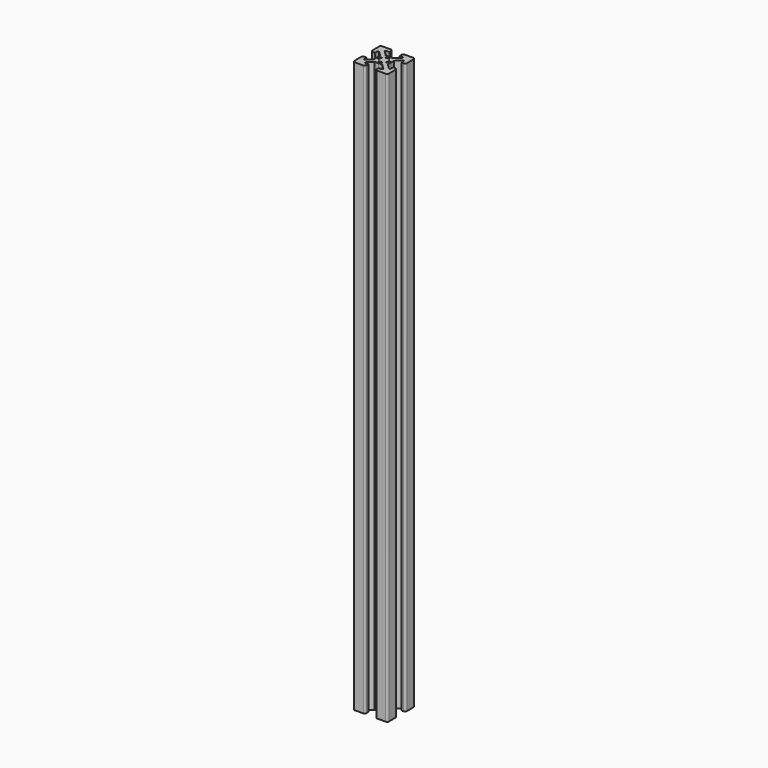
from build123d import *

# Parameters (mm, degrees)
F1_DEPTH = 330
F2_R     = 1
F3_R     = 0.5
F4_R     = 0.1


with BuildPart() as f1:
    # F0 (on Top) → F1 (new body)
    with BuildSketch(Plane.XY):
        with BuildLine():
            Line((-0.025, 4.0583112277), (-2.2905442747, 4.0583112277))
            Line((-2.2905442747, 4.0583112277), (-5.8640526549, 7.6318196079))
            Line((-5.8640526549, 7.6318196079), (-3, 7.6318196079))
            Line((-3, 7.6318196079), (-3, 10))
            Line((-3, 10), (-10, 10))
            Line((-10, 10), (-10, 3))
            Line((-10, 3), (-7.6318196079, 3))
            Line((-7.6318196079, 3), (-7.6318196079, 5.8640526549))
            Line((-7.6318196079, 5.8640526549), (-4, 2.232233047))
            Line((-4, 2.232233047), (-4, 0.025))
            Line((-4, 0.025), (-2.8230957687, 0.025))
            Line((-2.8230957687, 0.025), (-2.8230957687, 0.7926485917))
            Line((-2.8230957687, 0.7926485917), (-1.8740334308, 1.411684829))
            ThreePointArc((-1.8740334308, 1.411684829), (-2.3460869309, 0.0270456781), (-1.906078865, -1.3681077138))
            Line((-1.906078865, -1.3681077138), (-2.8238623803, -0.7794121329))
            Line((-2.8238623803, -0.7794121329), (-2.8238623803, -0.025))
            Line((-2.8238623803, -0.025), (-4, -0.025))
            Line((-4, -0.025), (-4, -2.232233047))
            Line((-4, -2.232233047), (-7.6318196079, -5.8640526549))
            Line((-7.6318196079, -5.8640526549), (-7.6318196079, -3))
            Line((-7.6318196079, -3), (-10, -3))
            Line((-10, -3), (-10, -10))
            Line((-10, -10), (-3, -10))
            Line((-3, -10), (-3, -7.6318196079))
            Line((-3, -7.6318196079), (-5.8640526549, -7.6318196079))
            Line((-5.8640526549, -7.6318196079), (-2.232233047, -4))
            Line((-2.232233047, -4), (-0.05, -4))
            Line((-0.05, -4), (-0.05, -2.9588690959))
            Line((-0.05, -2.9588690959), (-0.7483266194, -2.9588690959))
            Line((-0.7483266194, -2.9588690959), (-1.5537911294, -1.7580069631))
            ThreePointArc((-1.5537911294, -1.7580069631), (-0.0257632285, -2.3461013645), (1.5148107083, -1.7917041816))
            Line((1.5148107083, -1.7917041816), (0.7406048023, -2.9588690959))
            Line((0.7406048023, -2.9588690959), (0.05, -2.9588690959))
            Line((0.05, -2.9588690959), (0.05, -4))
            Line((0.05, -4), (2.232233047, -4))
            Line((2.232233047, -4), (5.8640526549, -7.6318196079))
            Line((5.8640526549, -7.6318196079), (3, -7.6318196079))
            Line((3, -7.6318196079), (3, -10))
            Line((3, -10), (10, -10))
            Line((10, -10), (10, -3))
            Line((10, -3), (7.6318196079, -3))
            Line((7.6318196079, -3), (7.6318196079, -5.8640526549))
            Line((7.6318196079, -5.8640526549), (4, -2.232233047))
            Line((4, -2.232233047), (4, -0.025))
            Line((4, -0.025), (2.8238623803, -0.025))
            Line((2.8238623803, -0.025), (2.8238623803, -0.7921485609))
            Line((2.8238623803, -0.7921485609), (1.8740334308, -1.411684829))
            ThreePointArc((1.8740334308, -1.411684829), (2.3460040432, 0.0334721598), (1.8329957125, 1.4645757318))
            Line((1.8329957125, 1.4645757318), (2.8230957687, 0.8068363719))
            Line((2.8230957687, 0.8068363719), (2.8230957687, 0.025))
            Line((2.8230957687, 0.025), (4, 0.025))
            Line((4, 0.025), (4, 2.232233047))
            Line((4, 2.232233047), (7.6318196079, 5.8640526549))
            Line((7.6318196079, 5.8640526549), (7.6318196079, 3))
            Line((7.6318196079, 3), (10, 3))
            Line((10, 3), (10, 10))
            Line((10, 10), (3, 10))
            Line((3, 10), (3, 7.6318196079))
            Line((3, 7.6318196079), (5.8640526549, 7.6318196079))
            Line((5.8640526549, 7.6318196079), (2.2905442747, 4.0583112277))
            Line((2.2905442747, 4.0583112277), (0.025, 4.0583112277))
            Line((0.025, 4.0583112277), (0.025, 2.9460287187))
            Line((0.025, 2.9460287187), (0.7554459771, 2.9460287187))
            Line((0.7554459771, 2.9460287187), (1.5118729288, 1.7941838266))
            ThreePointArc((1.5118729288, 1.7941838266), (-0.0195250931, 2.3461615731), (-1.5415243666, 1.7687730164))
            Line((-1.5415243666, 1.7687730164), (-0.7608180556, 2.9474266339))
            Line((-0.7608180556, 2.9474266339), (-0.025, 2.9474266339))
            Line((-0.025, 2.9474266339), (-0.025, 4.0583112277))
        make_face()
    extrude(amount=F1_DEPTH)

    # F2
    f2_edges = [f1.edges().sort_by_distance(p)[0] for p in [
        (10, 10, 165),
        (10, -10, 165),
        (-10, -10, 165),
        (-3, -10, 165),
        (3, -10, 165),
        (-3, 10, 165),
        (-10, 3, 165),
        (10, 3, 165),
        (10, -3, 165),
        (-10, -3, 165),
        (-10, 10, 165),
        (3, 10, 165),
    ]]
    fillet(f2_edges, radius=F2_R)

    # F3
    f3_edges = [f1.edges().sort_by_distance(p)[0] for p in [
        (-7.63182, 5.864053, 165),
        (-5.864053, 7.63182, 165),
        (5.864053, 7.63182, 165),
        (7.63182, 5.864053, 165),
        (-7.63182, -5.864053, 165),
        (-5.864053, -7.63182, 165),
        (5.864053, -7.63182, 165),
        (7.63182, -5.864053, 165),
    ]]
    fillet(f3_edges, radius=F3_R)

    # F4
    f4_edges = [f1.edges().sort_by_distance(p)[0] for p in [
        (-1.874033, 1.411685, 165),
        (2.290544, 4.058311, 165),
        (4.656946, 7.63182, 165),
        (-1.541524, 1.768773, 165),
        (1.514811, -1.791704, 165),
        (1.874033, -1.411685, 165),
        (1.832996, 1.464576, 165),
        (1.511873, 1.794184, 165),
        (-1.906079, -1.368108, 165),
        (-1.553791, -1.758007, 165),
    ]]
    fillet(f4_edges, radius=F4_R)


solid = f1.part
